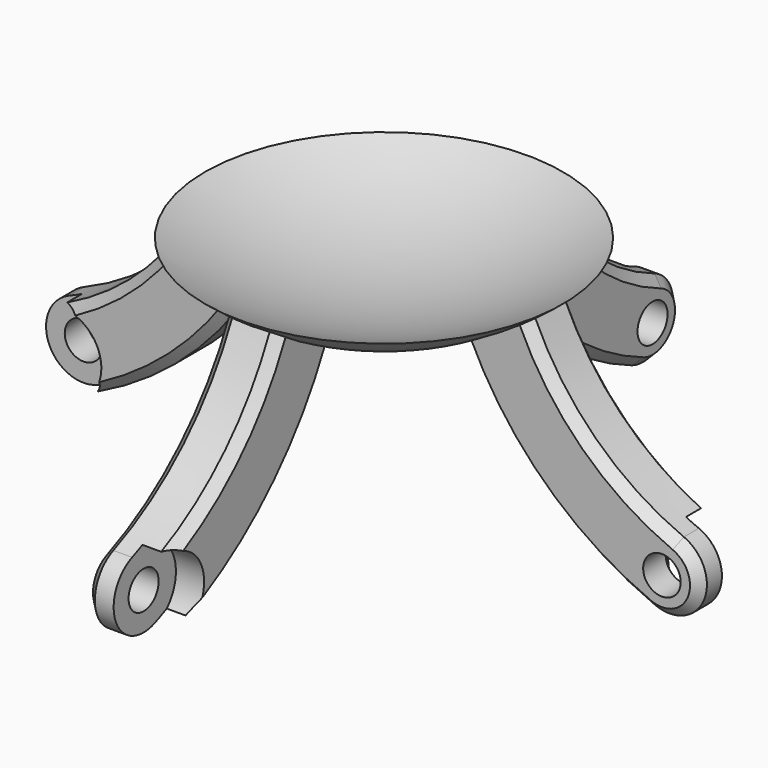
from build123d import *

# Parameters (mm, degrees)
F7_DEPTH         = 1.5
F7_COPIES_COUNT  = 4
F8_SIZE          = 0.5
F9_R             = 2.15
F10_DEPTH        = 1.5
F10_COPIES_COUNT = 4
F11_R            = 1
F12_DEPTH        = 3
F12_COPIES_COUNT = 4


# Not quite as in the source:
# - a pattern or mirror of a feature is missing from the dataset's text; its kind, count and spacing are read off the source's solid


with BuildPart() as f1:
    # F0 (on Top) → F1 (revolve)
    with BuildSketch(Plane.XY):
        with BuildLine():
            Line((0, -20), (0, 20))
            ThreePointArc((0, 20), (-20, 0), (0, -20))
        make_face()
    revolve(axis=Axis((0, 0, 0), (0, -1, 0)))

    # F2 (on Front) → F3 (revolve)
    with BuildSketch(Plane.XZ):
        with BuildLine():
            ThreePointArc((-4.5983759881, -20.2777777778), (-5.1275841713, -19.7652786452), (-5.6, -19.2))
            ThreePointArc((-5.6, -19.2), (-7.6082065121, -18.4963562268), (-9.5302879751, -17.5833333333))
            ThreePointArc((-9.5302879751, -17.5833333333), (-7.1916475208, -19.1635939597), (-4.5983759881, -20.2777777778))
        make_face()
        with BuildLine():
            Line((0, -21), (0, -20))
            ThreePointArc((0, -20), (-2.8284271247, -19.7989898732), (-5.6, -19.2))
            ThreePointArc((-5.6, -19.2), (-5.1275841713, -19.7652786452), (-4.5983759881, -20.2777777778))
            ThreePointArc((-4.5983759881, -20.2777777778), (-2.3273733406, -20.8183444869), (0, -21))
        make_face()
        with BuildLine():
            Line((0, -22), (0, -21))
            ThreePointArc((0, -21), (-2.3273733406, -20.8183444869), (-4.5983759881, -20.2777777778))
            ThreePointArc((-4.5983759881, -20.2777777778), (-2.4551533104, -21.5553201464), (0, -22))
        make_face()
    revolve(axis=Axis((0, 0, -21), (0, 0, -1)))

    # F4 (on Top) → F5 (revolve, cut)
    with BuildSketch(Plane.XY):
        with BuildLine():
            ThreePointArc((0, -20), (20, 0), (0, 20))
            Line((0, 20), (0, -20))
        make_face()
    revolve(axis=Axis((0, 0, 0), (0, -1, 0)), mode=Mode.SUBTRACT)

    # F6 (on Front) → F7 (join, symmetric)
    with BuildSketch(Plane.XZ):
        with BuildLine():
            ThreePointArc((16.7667947961, -25.7420411911), (12.0468652107, -22.6201202145), (8.8194778429, -17.9716692195))
            Line((8.8194778429, -17.9716692195), (5.3091861203, -19.8894418917))
            ThreePointArc((5.3091861203, -19.8894418917), (9.3769721823, -25.5877227261), (15.2332052039, -29.4246254756))
            ThreePointArc((15.2332052039, -29.4246254756), (17.8412921423, -28.3501281294), (16.7667947961, -25.7420411911))
        make_face()
    f7 = extrude(amount=F7_DEPTH, both=True)

    # F7_copies: F7 ×4 about axis
    f7_copies_axis = Axis((0, 0, 0), (0, 0, 1))
    for i in range(1, F7_COPIES_COUNT):
        add(f7.rotate(f7_copies_axis, i * 360 / F7_COPIES_COUNT))

    # F8
    f8_edges = [f1.edges().sort_by_distance(p)[0] for p in [
        (9.396954, 1.5, -25.606894),
        (17.841292, 1.5, -28.350128),
        (12.067102, 1.5, -22.639869),
        (12.067102, -1.5, -22.639869),
        (17.841292, -1.5, -28.350128),
        (9.396954, -1.5, -25.606894),
        (-12.067102, 1.5, -22.639869),
        (-12.067102, -1.5, -22.639869),
        (-9.396954, 1.5, -25.606894),
        (-17.841292, 1.5, -28.350128),
        (-9.396954, -1.5, -25.606894),
        (1.5, 9.396954, -25.606894),
        (-1.5, 9.396954, -25.606894),
        (1.5, 12.067102, -22.639869),
        (1.5, 17.841292, -28.350128),
        (-1.5, 12.067102, -22.639869),
        (-1.5, -9.396954, -25.606894),
        (1.5, -9.396954, -25.606894),
        (1.5, -12.067102, -22.639869),
        (-1.5, -12.067102, -22.639869),
        (-1.5, -17.841292, -28.350128),
    ]]
    chamfer(f8_edges, length=F8_SIZE)

    # F9 (on Front) → F10 (cut, through all)
    with BuildSketch(Plane.XZ):
        with Locations((16, -27.5833333333)):
            Circle(F9_R)
    f10 = extrude(amount=-F10_DEPTH, mode=Mode.SUBTRACT)

    # F10_copies: F10 ×4 about axis
    f10_copies_axis = Axis((0, 0, 0), (0, 0, 1))
    for i in range(1, F10_COPIES_COUNT):
        add(f10.rotate(f10_copies_axis, i * 360 / F10_COPIES_COUNT), mode=Mode.SUBTRACT)

    # F11 (on face) → F12 (cut, through all)
    with BuildSketch(Plane.XZ.offset(1.5)):
        with Locations((16, -27.5833333333)):
            Circle(F11_R)
    f12 = extrude(amount=-F12_DEPTH, mode=Mode.SUBTRACT)

    # F12_copies: F12 ×4 about axis
    f12_copies_axis = Axis((0, 0, 0), (0, 0, 1))
    for i in range(1, F12_COPIES_COUNT):
        add(f12.rotate(f12_copies_axis, i * 360 / F12_COPIES_COUNT), mode=Mode.SUBTRACT)


solid = f1.part
